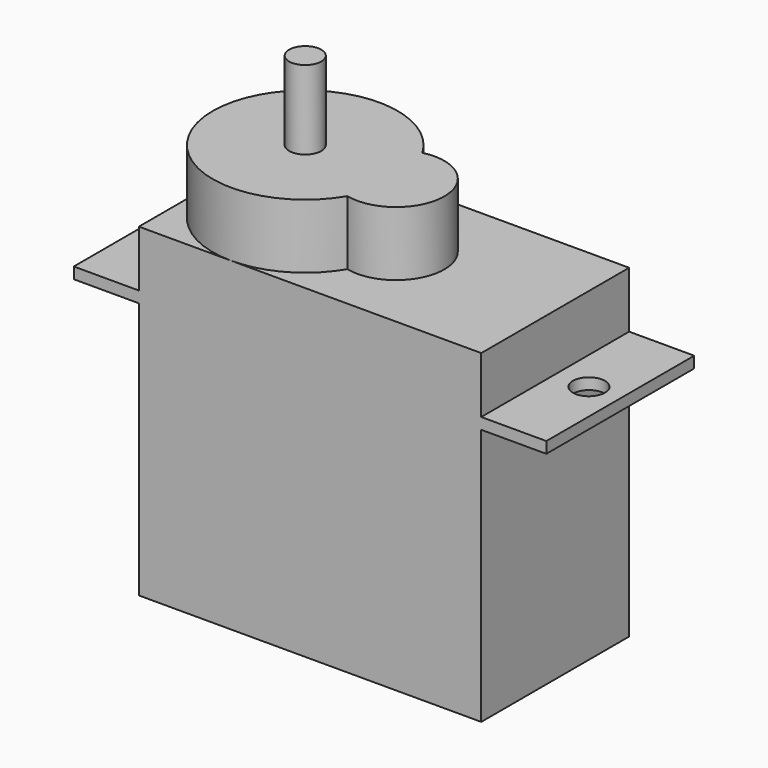
from build123d import *

# Parameters (mm, degrees)
F1_DEPTH = 11.5
F3_DEPTH = 4
F4_R     = 1
F5_DEPTH = 0.7
F6_R     = 1
F7_DEPTH = 0.7
F8_R     = 1
F9_DEPTH = 4.9


# Not quite as in the source:
# - a feature of the source that left no trace in its solid (it failed there, or was rolled back) is left out


with BuildPart() as f1:
    # F0 (on Front) → F1 (new body)
    with BuildSketch(Plane.XZ):
        Polygon((0, 16), (0, 0), (21.3, 0), (21.3, 16), (25.35, 16), (25.35, 16.7), (21.3, 16.7), (21.3, 20.2), (0, 20.2), (0, 16.7), (-4.05, 16.7), (-4.05, 16), align=None)
    extrude(amount=F1_DEPTH)

    # F2 (on face) → F3 (join)
    with BuildSketch(Plane.XY.offset(20.2)):
        with BuildLine():
            ThreePointArc((10.7044247788, -8.6682486377), (14.4, -5.75), (10.7044247788, -2.8317513623))
            ThreePointArc((10.7044247788, -2.8317513623), (0, -5.75), (10.7044247788, -8.6682486377))
        make_face()
    extrude(amount=F3_DEPTH)

    # F4 (on face) → F5 (cut, through all)
    with BuildSketch(Plane.XY.offset(16.7)):
        with Locations((-2.1, -5.75)):
            Circle(F4_R)
    extrude(amount=-F5_DEPTH, mode=Mode.SUBTRACT)

    # F6 (on face) → F7 (cut, through all)
    with BuildSketch(Plane.XY.offset(16.7)):
        with Locations((23.4, -5.75)):
            Circle(F6_R)
    extrude(amount=-F7_DEPTH, mode=Mode.SUBTRACT)

    # F8 (on face) → F9 (join)
    with BuildSketch(Plane.XY.offset(24.2)):
        with Locations((5.75, -5.75)):
            Circle(F8_R)
    extrude(amount=F9_DEPTH)


solid = f1.part
